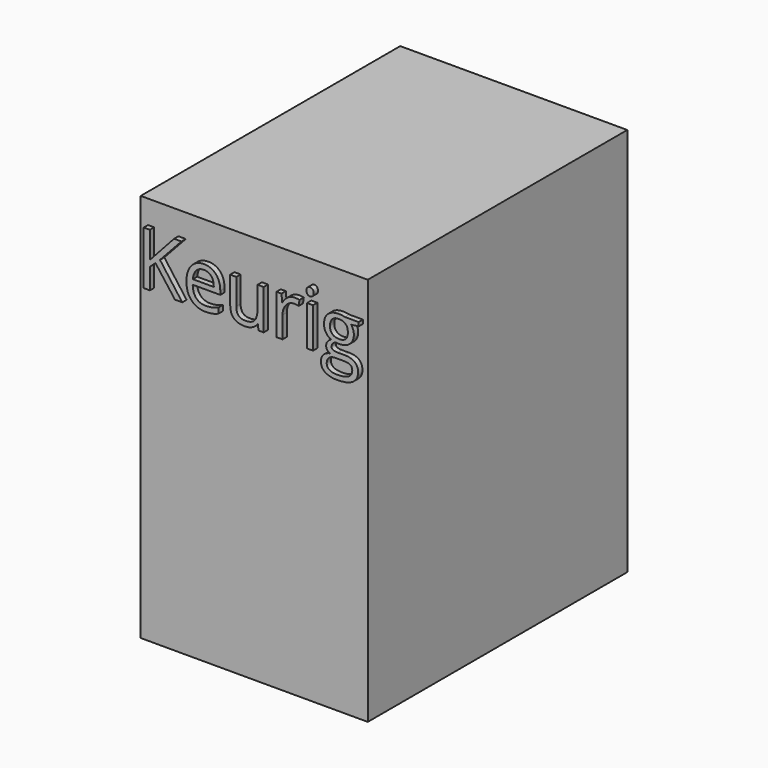
from build123d import *

# Parameters (mm, degrees)
F0_W         = 266.7
F0_H         = 457.2
F1_DEPTH     = 381
F2_TEXT_SIZE = 87.7708644007
F3_DEPTH     = 6.35


# Not quite as in the source:
# - Text() gives the source's letters only with a copy of the font that has no kerning and outlines rounded to 1/6400 em; it was checked with that copy


with BuildPart() as f1:
    # F0 (on Front) → F1 (new body)
    with BuildSketch(Plane.XZ):
        with Locations((133.35, 228.6)):
            Rectangle(F0_W, F0_H)
    extrude(amount=F1_DEPTH)

    # F2 (on face) → F3 (join)
    with BuildSketch(Plane.XZ.offset(381)):
        with Locations((0, 367.1998075565)):
            Text('Keurig', F2_TEXT_SIZE, font='Open Sans', text_align=(TextAlign.LEFT, TextAlign.BOTTOM))
    extrude(amount=F3_DEPTH)


solid = f1.part
